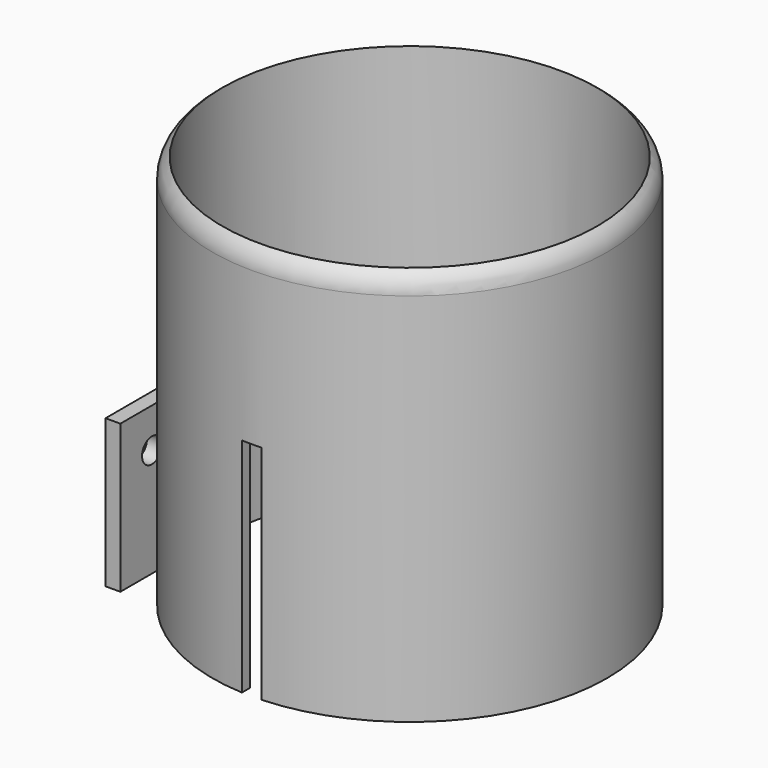
from build123d import *

# Parameters (mm, degrees)
F0_R      = 40
F1_DEPTH  = 80
F2_R      = 38
F3_DEPTH  = 90
F5_W      = 4
F5_H      = 45
F6_DEPTH  = 40
F7_W      = 3
F7_H      = 50
F8_DEPTH  = 30
F9_R      = 2.5
F10_DEPTH = 30


# Not quite as in the source:
# - a fillet or chamfer that OpenCascade refuses, or shapes differently, is made with other operations: its cross-section is extruded or revolved along the edge and cut away or added


with BuildPart() as f1:
    # F0 (on Top) → F1 (new body)
    with BuildSketch(Plane.XY):
        Circle(F0_R)
    extrude(amount=F1_DEPTH)

    # F2 (on face) → F3 (cut)
    with BuildSketch(Plane(origin=(0, 0, 0), x_dir=(1, 0, 0), z_dir=(0, 0, -1))):
        Circle(F2_R)
    extrude(amount=-F3_DEPTH, mode=Mode.SUBTRACT)

    # F4: fillet of radius 5 on 1 edges, made by hand

    # F4_s1 → F4_t2 (revolve, cut)
    with BuildSketch(Plane.XZ):
        with BuildLine():
            ThreePointArc((40, 76), (39.472135955, 78.2360679775), (38, 80))
            Line((38, 80), (40, 80))
            Line((40, 80), (40, 76))
        make_face()
    revolve(axis=Axis((0, 0, 80), (0, 0, 1)), mode=Mode.SUBTRACT)

    # F5 (on Front) → F6 (cut, symmetric)
    with BuildSketch(Plane.XZ):
        with Locations((-0.0568005547, 22.5)):
            Rectangle(F5_W, F5_H)
    extrude(amount=F6_DEPTH, both=True, mode=Mode.SUBTRACT)

    # F7 (on Top) → F8 (join)
    with BuildSketch(Plane.XY):
        with Locations((-40.154192288, 0)):
            Rectangle(F7_W, F7_H)
    extrude(amount=F8_DEPTH)

    # F9 (on face) → F10 (cut)
    with BuildSketch(Plane(origin=(-41.654192288, 0, 0), x_dir=(0, -1, 0), z_dir=(-1, 0, 0))):
        with Locations((-17, 22)):
            Circle(F9_R)
        with Locations((17, 22)):
            Circle(F9_R)
    extrude(amount=-F10_DEPTH, mode=Mode.SUBTRACT)


solid = f1.part
